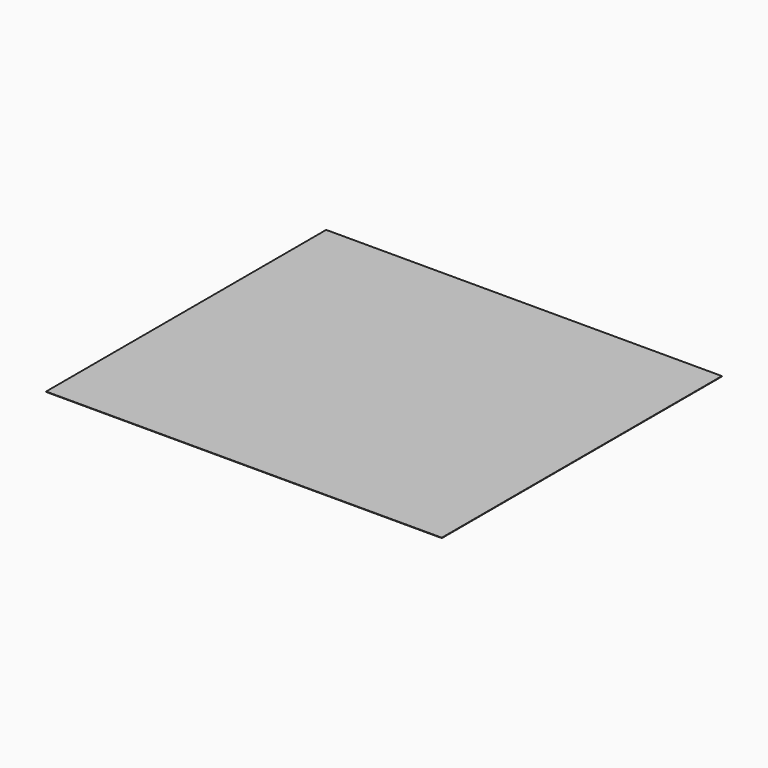
from build123d import *

# Parameters (mm, degrees)
F0_W     = 26000
F0_H     = 23000
F1_DEPTH = 25


# Not quite as in the source:
# - a feature names something its author has since deleted; it is built from what else it names


with BuildPart() as f1:
    # F0 (on Top) → F1 (new body)
    with BuildSketch(Plane.XY):
        with Locations((-13000, 11500)):
            Rectangle(F0_W, F0_H)
    extrude(amount=F1_DEPTH)


solid = f1.part
